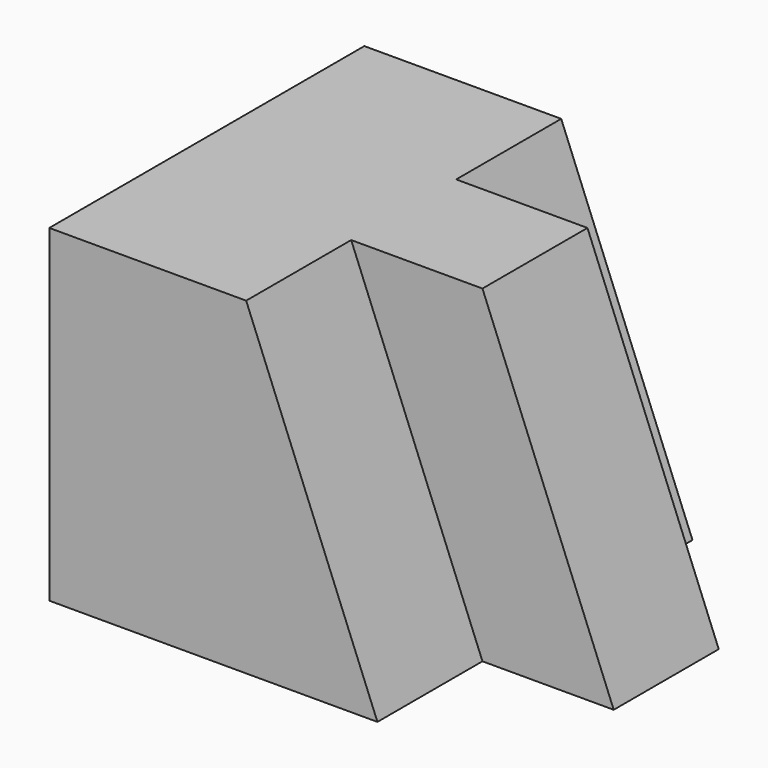
from build123d import *

# Parameters (mm, degrees)
F1_DEPTH = 31.75
F3_DEPTH = 25.401
F5_DEPTH = 12.7
F7_DEPTH = 12.7


# Not quite as in the source:
# - a length typed as a fraction of an inch, garbled in the dataset ("3 / 203.2 mm" for 3/8 in), is restored


with BuildPart() as f1:
    # F0 (on Top) → F1 (new body)
    with BuildSketch(Plane.XY):
        Polygon((-25.4, 38.1), (-44.45, 38.1), (-44.45, 0), (-25.4, 0), (-25.4, 12.7), (0, 12.7), (0, 25.4), (-25.4, 25.4), align=None)
    extrude(amount=F1_DEPTH)

    # F2 (on face) → F3 (cut, through all)
    with BuildSketch(Plane.XZ.offset(-12.7)):
        Polygon((0, 31.75), (-12.7, 31.75), (0, 0), align=None)
    extrude(amount=-F3_DEPTH, mode=Mode.SUBTRACT)

    # F4 (on face) → F5 (join)
    with BuildSketch(Plane.XZ.offset(-12.7)):
        Polygon((-12.7, 0), (-25.4, 31.75), (-25.4, 0), align=None)
    extrude(amount=F5_DEPTH)

    # F6 (on face) → F7 (join)
    with BuildSketch(Plane(origin=(0, 25.4, 0), x_dir=(-1, 0, 0), z_dir=(0, 1, 0))):
        Polygon((25.4, 0), (25.4, 31.75), (12.7, 0), align=None)
    extrude(amount=F7_DEPTH)


solid = f1.part
